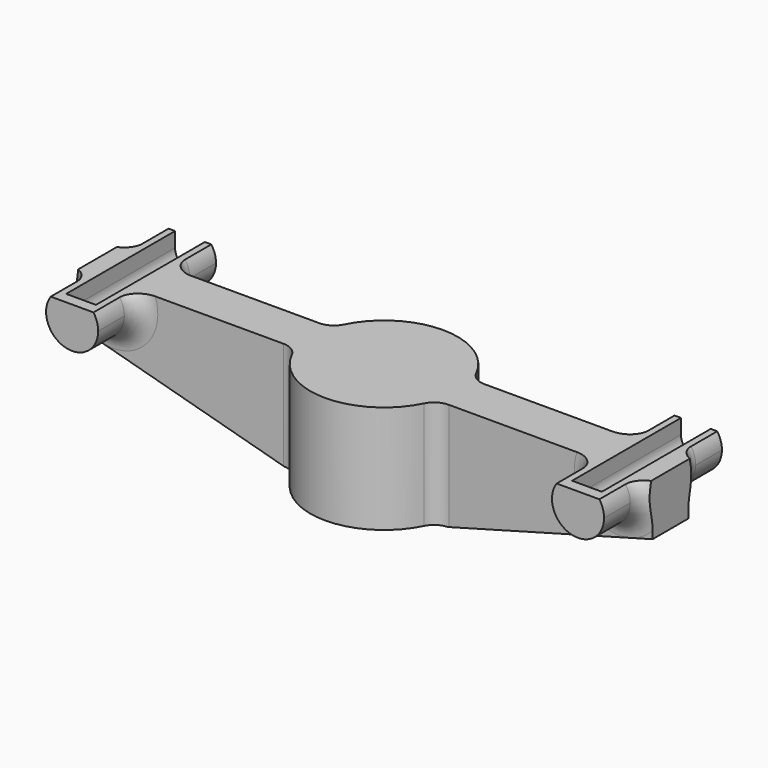
from build123d import *

# Parameters (mm, degrees)
F0_R           = 19.8
F0_R_2         = 16.8
F1_DEPTH       = 25
F2_R           = 19.8
F2_R_2         = 16.8
F3_DEPTH       = 4
F5_DEPTH       = 29
F6_SIZE2       = 55
F6_SIZE        = 15
F6_2_SIZE2     = 55
F6_2_SIZE      = 15
F7_R           = 5
F9_DEPTH       = 25
F10_DEPTH      = 13.8
F10_DEPTH_BACK = 25.8
F11_T4_ANGLE   = 359.64
F11_T10_ANGLE  = 359.64
F11_T16_ANGLE  = 359.64
F11_T22_ANGLE  = 359.64
F12_W          = 8
F12_H          = 8
F13_DEPTH      = 3


# Not quite as in the source:
# - a fillet or chamfer that OpenCascade refuses, or shapes differently, is made with other operations: its cross-section is extruded or revolved along the edge and cut away or added


with BuildPart() as f1:
    # F0 (on Top) → F1 (new body)
    with BuildSketch(Plane.XY):
        Circle(F0_R)
        Circle(F0_R_2, mode=Mode.SUBTRACT)
    extrude(amount=F1_DEPTH)

    # F2 (on face) → F3 (join)
    with BuildSketch(Plane.XY.offset(25)):
        Circle(F2_R)
        Circle(F2_R_2, mode=Mode.SUBTRACT)
        Circle(F2_R_2)
    extrude(amount=F3_DEPTH)

    # F4 (on face) → F5 (join)
    with BuildSketch(Plane.XY.offset(29)):
        with BuildLine():
            Line((-77, -6), (-18.8690222322, -6))
            ThreePointArc((-18.8690222322, -6), (-19.8, 0), (-18.8690222322, 6))
            Line((-18.8690222322, 6), (-77, 6))
            Line((-77, 6), (-77, -6))
        make_face()
        with BuildLine():
            Line((18.8690222322, -6), (77, -6))
            Line((77, -6), (77, 6))
            Line((77, 6), (18.8690222322, 6))
            ThreePointArc((18.8690222322, 6), (19.5658713095, 3.0358985327), (19.8, 0))
            ThreePointArc((19.8, 0), (19.5658713095, -3.0358985327), (18.8690222322, -6))
        make_face()
    extrude(amount=-F5_DEPTH)

    # F6
    f6_edges = [f1.edges().sort_by_distance(p)[0] for p in [
        (77, 0, 0),
    ]]
    f6_side = f1.faces().sort_by_distance((77, 0, 14.5))[0]
    chamfer(f6_edges, length=F6_SIZE, length2=F6_SIZE2, reference=f6_side)

    # F6#2
    f6_2_edges = [f1.edges().sort_by_distance(p)[0] for p in [
        (-77, 0, 0),
    ]]
    f6_2_side = f1.faces().sort_by_distance((-77, 0, 14.5))[0]
    chamfer(f6_2_edges, length=F6_2_SIZE, length2=F6_2_SIZE2, reference=f6_2_side)

    # F7 (call 1 of 4: OpenCascade refuses the feature's edges together)
    f7_edges = [f1.edges().sort_by_distance(p)[0] for p in [
        (-18.869022, 6, 14.5),
    ]]
    fillet(f7_edges, radius=F7_R)

    # F7#2 (call 2 of 4)
    f7_2_edges = [f1.edges().sort_by_distance(p)[0] for p in [
        (18.869022, 6, 14.5),
    ]]
    fillet(f7_2_edges, radius=F7_R)

    # F7#3 (call 3 of 4)
    f7_3_edges = [f1.edges().sort_by_distance(p)[0] for p in [
        (-18.869022, -6, 14.5),
    ]]
    fillet(f7_3_edges, radius=F7_R)

    # F7#4 (call 4 of 4)
    f7_4_edges = [f1.edges().sort_by_distance(p)[0] for p in [
        (18.869022, -6, 14.5),
    ]]
    fillet(f7_4_edges, radius=F7_R)

    # F8 (on face) → F9 (cut)
    with BuildSketch(Plane.XZ.offset(6)):
        with BuildLine():
            ThreePointArc((68, 29), (70.8284271247, 27.8284271247), (72, 25))
            Line((72, 25), (72, 29))
            Line((72, 29), (68, 29))
        make_face()
        with BuildLine():
            Line((64, 29), (64, 25))
            ThreePointArc((64, 25), (65.1715728753, 27.8284271247), (68, 29))
            Line((68, 29), (64, 29))
        make_face()
        with BuildLine():
            ThreePointArc((68, 29), (65.1715728753, 27.8284271247), (64, 25))
            ThreePointArc((64, 25), (68, 21), (72, 25))
            ThreePointArc((72, 25), (70.8284271247, 27.8284271247), (68, 29))
        make_face()
        with BuildLine():
            Line((-72, 29), (-72, 25))
            ThreePointArc((-72, 25), (-70.8284271247, 27.8284271247), (-68, 29))
            Line((-68, 29), (-72, 29))
        make_face()
        with BuildLine():
            ThreePointArc((-68, 29), (-65.1715728753, 27.8284271247), (-64, 25))
            Line((-64, 25), (-64, 29))
            Line((-64, 29), (-68, 29))
        make_face()
        with BuildLine():
            ThreePointArc((-68, 29), (-70.8284271247, 27.8284271247), (-72, 25))
            ThreePointArc((-72, 25), (-68, 21), (-64, 25))
            ThreePointArc((-64, 25), (-65.1715728753, 27.8284271247), (-68, 29))
        make_face()
    extrude(amount=-F9_DEPTH, mode=Mode.SUBTRACT)

    # F8 (on face) → F10 (join, two sides)
    with BuildSketch(Plane.XZ.offset(6)) as f10_sk:
        with BuildLine():
            ThreePointArc((-64, 25), (-68, 21), (-72, 25))
            Line((-72, 25), (-72, 29))
            Line((-72, 29), (-73.7445626465, 29))
            ThreePointArc((-73.7445626465, 29), (-70.0961943462, 18.3212299588), (-61, 25))
            ThreePointArc((-61, 25), (-61.3212299588, 27.0961943462), (-62.2554373535, 29))
            Line((-62.2554373535, 29), (-64, 29))
            Line((-64, 29), (-64, 25))
        make_face()
        with BuildLine():
            ThreePointArc((72, 25), (68, 21), (64, 25))
            Line((64, 25), (64, 29))
            Line((64, 29), (62.2554373535, 29))
            ThreePointArc((62.2554373535, 29), (65.9038056538, 18.3212299588), (75, 25))
            ThreePointArc((75, 25), (74.6787700412, 27.0961943462), (73.7445626465, 29))
            Line((73.7445626465, 29), (72, 29))
            Line((72, 29), (72, 25))
        make_face()
    extrude(amount=F10_DEPTH)
    extrude(f10_sk.sketch, amount=-F10_DEPTH_BACK)

    # F11: fillet of radius 5 on 4 edges, made by hand


with BuildPart() as f11_tool2:
    # F11_s3 → F11_t4 (revolve)
    with BuildSketch(Plane(origin=(67.9207895695, 0, -0.2133801555), x_dir=(0, 1, 0), z_dir=(-0.9999950652, 0, 0.0031415875))):
        with BuildLine():
            ThreePointArc((6, -37.2135045791), (7.4644660941, -33.6779706732), (11, -32.2135045791))
            Line((11, -32.2135045791), (6, -32.2135045791))
            Line((6, -32.2135045791), (6, -37.2135045791))
        make_face()
    revolve(axis=Axis((68, 6, 25), (0, 1, 0)), revolution_arc=F11_T4_ANGLE)

    split(bisect_by=Plane.XY.offset(29), keep=Keep.BOTTOM)

    split(bisect_by=Plane.YZ.offset(77), keep=Keep.BOTTOM)


with BuildPart() as f1_1:
    add(f1.part)

    # F11_t1: union F11_tool2
    add(f11_tool2.part)


with BuildPart() as f11_tool8:
    # F11_s9 → F11_t10 (revolve)
    with BuildSketch(Plane(origin=(67.9207895695, 0, -0.2133801555), x_dir=(0, 1, 0), z_dir=(-0.9999950652, 0, 0.0031415875))):
        with BuildLine():
            ThreePointArc((-11, -32.2135045791), (-7.4644660941, -33.6779706732), (-6, -37.2135045791))
            Line((-6, -37.2135045791), (-6, -32.2135045791))
            Line((-6, -32.2135045791), (-11, -32.2135045791))
        make_face()
    revolve(axis=Axis((68, -6, 25), (0, 1, 0)), revolution_arc=F11_T10_ANGLE)

    split(bisect_by=Plane.XY.offset(29), keep=Keep.BOTTOM)

    split(bisect_by=Plane.YZ.offset(77), keep=Keep.BOTTOM)


with BuildPart() as f1_2:
    add(f1_1.part)

    # F11_t7: union F11_tool8
    add(f11_tool8.part)


with BuildPart() as f11_tool14:
    # F11_s15 → F11_t16 (revolve)
    with BuildSketch(Plane(origin=(-68.0778681687, 0, 0.2138736341), x_dir=(0, 1, 0), z_dir=(-0.9999950652, 0, 0.0031415875))):
        with BuildLine():
            ThreePointArc((11, -31.786248681), (7.4644660941, -33.2507147751), (6, -36.786248681))
            Line((6, -36.786248681), (6, -31.786248681))
            Line((6, -31.786248681), (11, -31.786248681))
        make_face()
    revolve(axis=Axis((-68, 6, 25), (0, 1, 0)), revolution_arc=F11_T16_ANGLE)

    split(bisect_by=Plane.XY.offset(29), keep=Keep.BOTTOM)

    split(bisect_by=Plane.YZ.offset(-77), keep=Keep.TOP)


with BuildPart() as f1_3:
    add(f1_2.part)

    # F11_t13: union F11_tool14
    add(f11_tool14.part)


with BuildPart() as f11_tool20:
    # F11_s21 → F11_t22 (revolve)
    with BuildSketch(Plane(origin=(-68.0778681687, 0, 0.2138736341), x_dir=(0, 1, 0), z_dir=(-0.9999950652, 0, 0.0031415875))):
        with BuildLine():
            ThreePointArc((-6, -36.786248681), (-7.4644660941, -33.2507147751), (-11, -31.786248681))
            Line((-11, -31.786248681), (-6, -31.786248681))
            Line((-6, -31.786248681), (-6, -36.786248681))
        make_face()
    revolve(axis=Axis((-68, -6, 25), (0, 1, 0)), revolution_arc=F11_T22_ANGLE)

    split(bisect_by=Plane.XY.offset(29), keep=Keep.BOTTOM)

    split(bisect_by=Plane.YZ.offset(-77), keep=Keep.TOP)


with BuildPart() as f1_4:
    add(f1_3.part)

    # F11_t19: union F11_tool20
    add(f11_tool20.part)

    # F12 (on face) → F13 (join)
    with BuildSketch(Plane.XZ.offset(19.8)):
        with Locations((68, 25)):
            Rectangle(F12_W, F12_H)
        with BuildLine():
            Line((-64, 29), (-72, 29))
            Line((-72, 29), (-72, 25))
            ThreePointArc((-72, 25), (-70.8284271247, 22.1715728753), (-68, 21))
            ThreePointArc((-68, 21), (-65.1715728753, 22.1715728753), (-64, 25))
            Line((-64, 25), (-64, 29))
        make_face()
        with BuildLine():
            Line((-64, 21), (-64, 25))
            ThreePointArc((-64, 25), (-65.1715728753, 22.1715728753), (-68, 21))
            Line((-68, 21), (-64, 21))
        make_face()
        with BuildLine():
            ThreePointArc((-68, 21), (-70.8284271247, 22.1715728753), (-72, 25))
            Line((-72, 25), (-72, 21))
            Line((-72, 21), (-68, 21))
        make_face()
    extrude(amount=-F13_DEPTH)


solid = f1_4.part
